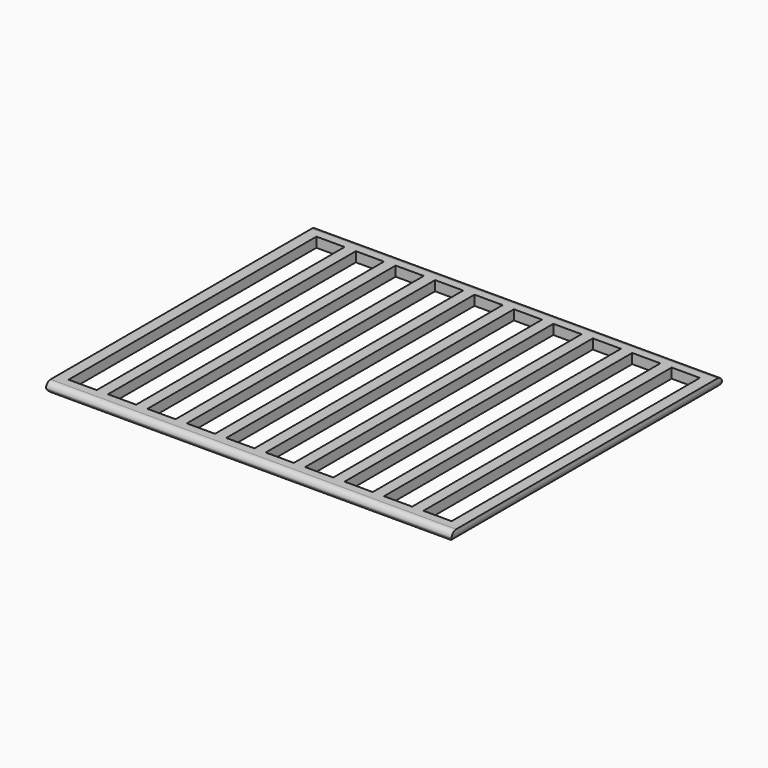
from build123d import *

# Parameters (mm, degrees)
F0_W        = 144
F0_H        = 120
F0_W_2      = 10
F0_H_2      = 110
F0_H_3      = 110.1521776617
F0_H_4      = 110.1521739364
F1_DEPTH    = 3.5
F2_R        = 2
F3_T1_DEPTH = 153.6824583655
F4_T1_DEPTH = 126.1270166538


# Not quite as in the source:
# - a fillet or chamfer that OpenCascade refuses, or shapes differently, is made with other operations: its cross-section is extruded or revolved along the edge and cut away or added


with BuildPart() as f1:
    # F0 (on Top) → F1 (new body)
    with BuildSketch(Plane.XY):
        Rectangle(F0_W, F0_H)
        with Locations((-63, 0)):
            Rectangle(F0_W_2, F0_H_2, mode=Mode.SUBTRACT)
        with Locations((-49, 0)):
            Rectangle(F0_W_2, F0_H_2, mode=Mode.SUBTRACT)
        with Locations((-35, 0.0760888308)):
            Rectangle(F0_W_2, F0_H_3, mode=Mode.SUBTRACT)
        with Locations((-21, 0.0760869682)):
            Rectangle(F0_W_2, F0_H_4, mode=Mode.SUBTRACT)
        with Locations((-7, 0.0760869682)):
            Rectangle(F0_W_2, F0_H_4, mode=Mode.SUBTRACT)
        with Locations((7, 0.0760869682)):
            Rectangle(F0_W_2, F0_H_4, mode=Mode.SUBTRACT)
        with Locations((21, 0.0760888308)):
            Rectangle(F0_W_2, F0_H_3, mode=Mode.SUBTRACT)
        with Locations((35, 0.0760869682)):
            Rectangle(F0_W_2, F0_H_4, mode=Mode.SUBTRACT)
        with Locations((49, 0.0760888308)):
            Rectangle(F0_W_2, F0_H_3, mode=Mode.SUBTRACT)
        with Locations((63, 0.0760888308)):
            Rectangle(F0_W_2, F0_H_3, mode=Mode.SUBTRACT)
    extrude(amount=F1_DEPTH)

    # F2
    f2_edges = [f1.edges().sort_by_distance(p)[0] for p in [
        (0, 60, 3.5),
        (0, -60, 3.5),
    ]]
    fillet(f2_edges, radius=F2_R)

    # F3: fillet of radius 2 on 2 edges, made by hand

    # F3_s2 → F3_t1 (cut)
    with BuildSketch(Plane.YZ.offset(-76.8412291828)):
        with BuildLine():
            ThreePointArc((-58.0635083269, 0), (-59.2882531983, 0.4188611699), (-60, 1.5))
            Line((-60, 1.5), (-60, 0))
            Line((-60, 0), (-58.0635083269, 0))
        make_face()
        with BuildLine():
            ThreePointArc((60, 1.5), (59.2882531983, 0.4188611699), (58.0635083269, 0))
            Line((58.0635083269, 0), (60, 0))
            Line((60, 0), (60, 1.5))
        make_face()
    extrude(amount=F3_T1_DEPTH, mode=Mode.SUBTRACT)

    # F4: fillet of radius 2 on 2 edges, made by hand

    # F4_s2 → F4_t1 (cut)
    with BuildSketch(Plane.XZ.offset(-63.0635083269)):
        with BuildLine():
            ThreePointArc((-72, 2), (-71.4142135624, 0.5857864376), (-70, 0))
            Line((-70, 0), (-72, 0))
            Line((-72, 0), (-72, 2))
        make_face()
        with BuildLine():
            ThreePointArc((72, 2), (71.4142135624, 0.5857864376), (70, 0))
            Line((70, 0), (72, 0))
            Line((72, 0), (72, 2))
        make_face()
    extrude(amount=F4_T1_DEPTH, mode=Mode.SUBTRACT)


solid = f1.part
